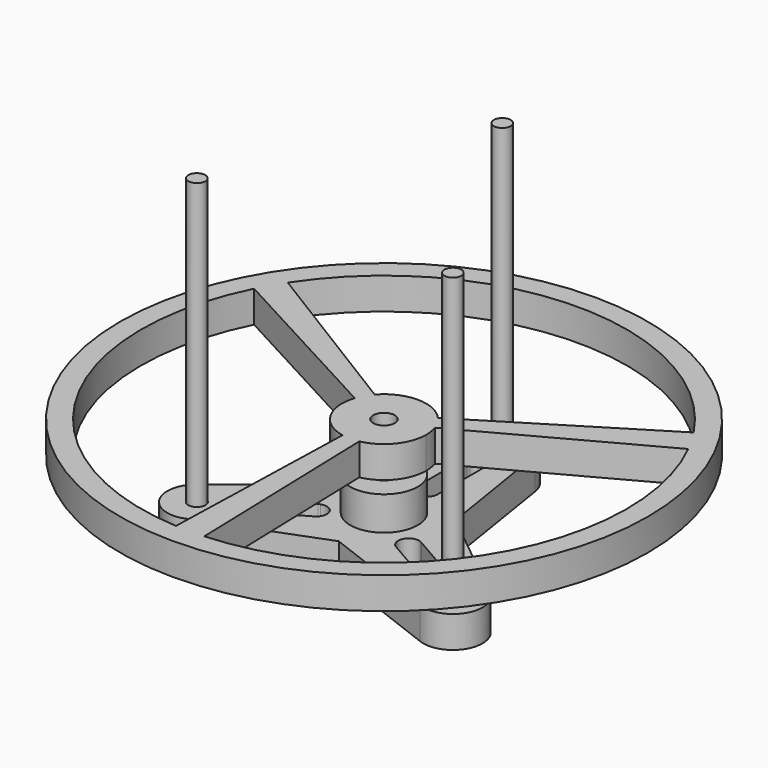
from build123d import *

# Parameters (mm, degrees)
F0_R      = 4
F1_DEPTH  = 150
F2_R      = 4.1
F3_DEPTH  = 15
F5_R      = 125
F6_DEPTH  = 15
F7_D      = 10.2
F9_R      = 16
F10_DEPTH = 16
F11_R     = 5
F12_DEPTH = 15


# Not quite as in the source:
# - a feature names something its author has since deleted; it is built from what else it names


with BuildPart() as f1:
    # F0 (on Top) → F1 (new body)
    with BuildSketch(Plane.XY):
        with Locations((0, 70)):
            Circle(F0_R)
    extrude(amount=F1_DEPTH)


with BuildPart() as f1b:
    # F0 (on Top) → F1, piece 2 (new body)
    with BuildSketch(Plane.XY):
        with Locations((-60.6217782649, -35)):
            Circle(F0_R)
    extrude(amount=F1_DEPTH)


with BuildPart() as f1c:
    # F0 (on Top) → F1, piece 3 (new body)
    with BuildSketch(Plane.XY):
        with Locations((60.6217782649, -35)):
            Circle(F0_R)
    extrude(amount=F1_DEPTH)


with BuildPart() as f3:
    # F2 (on Top) → F3 (new body)
    with BuildSketch(Plane.XY):
        with BuildLine():
            ThreePointArc((-15.7469411811, 19.4173593323), (-10.6083266094, 22.6376546168), (-4.8455068732, 24.5259263462))
            ThreePointArc((-4.8455068732, 24.5259263462), (-4.8928885521, 24.9209603499), (-4.9087158404, 25.3185108304))
            Line((-4.9087158404, 25.3185108304), (-4.9087158404, 55.3185108304))
            ThreePointArc((-4.9087158404, 55.3185108304), (-4.851787509, 56.0709261545), (-4.6822986521, 56.8062105772))
            ThreePointArc((-4.6822986521, 56.8062105772), (-12.0366957637, 62.8503178328), (-13.8260623462, 72.2))
            Line((-13.8260623462, 72.2), (-23.1845919064, 13.3856303782))
            Line((-23.1845919064, 13.3856303782), (-15.7469411811, 19.4173593323))
        make_face()
        with BuildLine():
            ThreePointArc((14, 70), (13.956447844, 71.1034326336), (13.8260623462, 72.2))
            ThreePointArc((13.8260623462, 72.2), (0, 84), (-13.8260623462, 72.2))
            ThreePointArc((-13.8260623462, 72.2), (-12.0366957637, 62.8503178328), (-4.6822986521, 56.8062105772))
            ThreePointArc((-4.6822986521, 56.8062105772), (0.0606919076, 60.3191708855), (4.8473554351, 56.865954725))
            ThreePointArc((4.8473554351, 56.865954725), (11.486143306, 61.9957191482), (14, 70))
        make_face()
        with Locations((0, 70)):
            Circle(F2_R, mode=Mode.SUBTRACT)
        with BuildLine():
            ThreePointArc((5.0236987184, 24.4900480029), (10.6905525136, 22.598939952), (15.7469411811, 19.4173593323))
            Line((15.7469411811, 19.4173593323), (23.1845919064, 13.3856303782))
            Line((23.1845919064, 13.3856303782), (13.8260623462, 72.2))
            ThreePointArc((13.8260623462, 72.2), (13.956447844, 71.1034326336), (14, 70))
            ThreePointArc((14, 70), (11.486143306, 61.9957191482), (4.8473554351, 56.865954725))
            ThreePointArc((4.8473554351, 56.865954725), (5.0210368519, 56.1626662615), (5.0912841596, 55.4416633397))
            Line((5.0912841596, 55.4416633397), (5.0912841596, 25.4416633397))
            ThreePointArc((5.0912841596, 25.4416633397), (5.0802361713, 24.9642402993), (5.0236987184, 24.4900480029))
        make_face()
        with BuildLine():
            ThreePointArc((23.6628287038, -8.0666311267), (24.6634417468, -4.0883543391), (25, 0))
            ThreePointArc((25, 0), (24.9222282929, 1.9704154171), (24.6893970467, 3.9285714286))
            ThreePointArc((24.6893970467, 3.9285714286), (21.6506350946, 12.5), (15.7469411811, 19.4173593323))
            ThreePointArc((15.7469411811, 19.4173593323), (10.6905525136, 22.598939952), (5.0236987184, 24.4900480029))
            ThreePointArc((5.0236987184, 24.4900480029), (0.0738629344, 20.3177855481), (-4.8455068732, 24.5259263462))
            ThreePointArc((-4.8455068732, 24.5259263462), (-10.6083266094, 22.6376546168), (-15.7469411811, 19.4173593323))
            ThreePointArc((-15.7469411811, 19.4173593323), (-21.6506350946, 12.5), (-24.6893970467, 3.9285714286))
            ThreePointArc((-24.6893970467, 3.9285714286), (-24.9165323538, -2.0411799187), (-23.7208530697, -7.8943732904))
            ThreePointArc((-23.7208530697, -7.8943732904), (-17.6326499005, -10.0949255965), (-18.8173218306, -16.4592952196))
            ThreePointArc((-18.8173218306, -16.4592952196), (-14.3006206755, -20.5059076438), (-8.9424558656, -23.3459307609))
            ThreePointArc((-8.9424558656, -23.3459307609), (0, -25), (8.9424558656, -23.3459307609))
            ThreePointArc((8.9424558656, -23.3459307609), (14.2259798402, -20.5577600333), (18.6971543512, -16.5956747126))
            ThreePointArc((18.6971543512, -16.5956747126), (17.5587869661, -10.2228599516), (23.6628287038, -8.0666311267))
        make_face()
        with BuildLine():
            Line((-24.6893970467, 3.9285714286), (-23.1845919064, 13.3856303782))
            Line((-23.1845919064, 13.3856303782), (-69.4400653263, -24.1262787739))
            ThreePointArc((-69.4400653263, -24.1262787739), (-60.5360847426, -21.000262266), (-51.6710391199, -24.2350444145))
            ThreePointArc((-51.6710391199, -24.2350444145), (-51.1488141527, -23.7329876636), (-50.5595309601, -23.3116502498))
            Line((-50.5595309601, -23.3116502498), (-24.5787688465, -8.3116502498))
            ThreePointArc((-24.5787688465, -8.3116502498), (-24.1597843711, -8.0825065681), (-23.7208530697, -7.8943732904))
            ThreePointArc((-23.7208530697, -7.8943732904), (-24.9165323538, -2.0411799187), (-24.6893970467, 3.9285714286))
        make_face()
        with BuildLine():
            ThreePointArc((-69.4400653263, -24.1262787739), (-72.7461339179, -42), (-55.6140029802, -48.0737212261))
            ThreePointArc((-55.6140029802, -48.0737212261), (-49.0868562022, -42.9338246141), (-46.6217782649, -35))
            ThreePointArc((-46.6217782649, -35), (-46.6800730977, -33.723733166), (-46.8544721266, -32.4580948694))
            ThreePointArc((-46.8544721266, -32.4580948694), (-52.2682802758, -30.107024709), (-51.6710391199, -24.2350444145))
            ThreePointArc((-51.6710391199, -24.2350444145), (-60.5360847426, -21.000262266), (-69.4400653263, -24.1262787739))
        make_face()
        with Locations((-60.6217782649, -35)):
            Circle(F2_R, mode=Mode.SUBTRACT)
        with BuildLine():
            Line((0, -26.7712607564), (-8.9424558656, -23.3459307609))
            ThreePointArc((-8.9424558656, -23.3459307609), (-14.3006206755, -20.5059076438), (-18.8173218306, -16.4592952196))
            ThreePointArc((-18.8173218306, -16.4592952196), (-19.1357404737, -16.697845959), (-19.4721156449, -16.910328033))
            Line((-19.4721156449, -16.910328033), (-45.4528777584, -31.910328033))
            ThreePointArc((-45.4528777584, -31.910328033), (-46.132952709, -32.2372343138), (-46.8544721266, -32.4580948694))
            ThreePointArc((-46.8544721266, -32.4580948694), (-46.6800730977, -33.723733166), (-46.6217782649, -35))
            ThreePointArc((-46.6217782649, -35), (-49.0868562022, -42.9338246141), (-55.6140029802, -48.0737212261))
            Line((-55.6140029802, -48.0737212261), (0, -26.7712607564))
        make_face()
        with BuildLine():
            ThreePointArc((19.487484687, -17.1300130899), (19.0795481998, -16.8817337312), (18.6971543512, -16.5956747126))
            ThreePointArc((18.6971543512, -16.5956747126), (14.2259798402, -20.5577600333), (8.9424558656, -23.3459307609))
            Line((8.9424558656, -23.3459307609), (0, -26.7712607564))
            Line((0, -26.7712607564), (55.6140029802, -48.0737212261))
            ThreePointArc((55.6140029802, -48.0737212261), (48.4548029798, -41.9256560998), (46.8236836847, -32.6309103105))
            ThreePointArc((46.8236836847, -32.6309103105), (46.1277773008, -32.4296785979), (45.4682468005, -32.1300130899))
            Line((45.4682468005, -32.1300130899), (19.487484687, -17.1300130899))
        make_face()
        with BuildLine():
            ThreePointArc((24.6893970467, 3.9285714286), (24.9222282929, 1.9704154171), (25, 0))
            ThreePointArc((25, 0), (24.6634417468, -4.0883543391), (23.6628287038, -8.0666311267))
            ThreePointArc((23.6628287038, -8.0666311267), (24.0286290258, -8.2231143909), (24.3808314853, -8.4081827974))
            Line((24.3808314853, -8.4081827974), (50.3615935989, -23.4081827974))
            ThreePointArc((50.3615935989, -23.4081827974), (50.984740218, -23.8336918407), (51.5367707787, -24.3481157078))
            ThreePointArc((51.5367707787, -24.3481157078), (60.448319761, -21.0010746074), (69.4400653263, -24.1262787739))
            Line((69.4400653263, -24.1262787739), (23.1845919064, 13.3856303782))
            Line((23.1845919064, 13.3856303782), (24.6893970467, 3.9285714286))
        make_face()
        with BuildLine():
            ThreePointArc((74.6217782649, -35), (73.2601329612, -28.97737677), (69.4400653263, -24.1262787739))
            ThreePointArc((69.4400653263, -24.1262787739), (60.448319761, -21.0010746074), (51.5367707787, -24.3481157078))
            ThreePointArc((51.5367707787, -24.3481157078), (52.2075883683, -30.2121461765), (46.8236836847, -32.6309103105))
            ThreePointArc((46.8236836847, -32.6309103105), (48.4548029798, -41.9256560998), (55.6140029802, -48.0737212261))
            ThreePointArc((55.6140029802, -48.0737212261), (68.555602879, -46.5349220627), (74.6217782649, -35))
        make_face()
        with Locations((60.6217782649, -35)):
            Circle(F2_R, mode=Mode.SUBTRACT)
        with BuildLine():
            ThreePointArc((15.7469411811, 19.4173593323), (21.6506350946, 12.5), (24.6893970467, 3.9285714286))
            Line((24.6893970467, 3.9285714286), (23.1845919064, 13.3856303782))
            Line((23.1845919064, 13.3856303782), (15.7469411811, 19.4173593323))
        make_face()
        with BuildLine():
            ThreePointArc((-24.6893970467, 3.9285714286), (-21.6506350946, 12.5), (-15.7469411811, 19.4173593323))
            Line((-15.7469411811, 19.4173593323), (-23.1845919064, 13.3856303782))
            Line((-23.1845919064, 13.3856303782), (-24.6893970467, 3.9285714286))
        make_face()
        with BuildLine():
            Line((0, -26.7712607564), (8.9424558656, -23.3459307609))
            ThreePointArc((8.9424558656, -23.3459307609), (0, -25), (-8.9424558656, -23.3459307609))
            Line((-8.9424558656, -23.3459307609), (0, -26.7712607564))
        make_face()
    extrude(amount=F3_DEPTH)


with BuildPart() as f6:
    # F5 (on offset) → F6 (new body)
    with BuildSketch(Plane.XY.offset(40)):
        Circle(F5_R)
        with BuildLine():
            ThreePointArc((102.7583822566, 51.6305614534), (111.8977523445, 26.5309822706), (115, 0))
            ThreePointArc((115, 0), (83.6577855811, -78.9073818579), (6.7152189274, -114.8037709954))
            ThreePointArc((6.7152189274, -114.8037709954), (0.0247447273, -114.9999973378), (-6.665813298, -114.8066502128))
            ThreePointArc((-6.665813298, -114.8066502128), (-99.5805467661, -57.5214282313), (-102.7805915959, 51.5863353146))
            ThreePointArc((-102.7805915959, 51.5863353146), (-99.6052914933, 57.4785691065), (-96.0925689586, 63.1760887593))
            ThreePointArc((-96.0925689586, 63.1760887593), (-0.0247447273, 114.9999973378), (96.0653726685, 63.2174356808))
            ThreePointArc((96.0653726685, 63.2174356808), (99.5805467661, 57.5214282313), (102.7583822566, 51.6305614534))
        make_face(mode=Mode.SUBTRACT)
        with BuildLine():
            Line((-14.9932737383, 13.2363795129), (-96.0925689586, 63.1760887593))
            ThreePointArc((-96.0925689586, 63.1760887593), (-99.6052914933, 57.4785691065), (-102.7805915959, 51.5863353146))
            Line((-102.7805915959, 51.5863353146), (-18.9593623085, 6.3673056198))
            ThreePointArc((-18.9593623085, 6.3673056198), (-17.3202603233, 10.0004291074), (-14.9932737383, 13.2363795129))
        make_face()
        with BuildLine():
            Line((18.9596777814, 6.3663661868), (102.7583822566, 51.6305614534))
            ThreePointArc((102.7583822566, 51.6305614534), (99.5805467661, 57.5214282313), (96.0653726685, 63.2174356808))
            Line((96.0653726685, 63.2174356808), (14.9939295747, 13.2356365888))
            ThreePointArc((14.9939295747, 13.2356365888), (17.3207558174, 9.9995708864), (18.9596777814, 6.3663661868))
        make_face()
        with BuildLine():
            ThreePointArc((-6.665813298, -114.8066502128), (0.0247447273, -114.9999973378), (6.7152189274, -114.8037709954))
            Line((6.7152189274, -114.8037709954), (3.9654327338, -19.6029422086))
            ThreePointArc((3.9654327338, -19.6029422086), (-0.0004954941, -19.9999999939), (-3.9664040432, -19.6027456997))
            Line((-3.9664040432, -19.6027456997), (-6.665813298, -114.8066502128))
        make_face()
        with BuildLine():
            ThreePointArc((20, 0), (19.7382060435, 3.2254026393), (18.9596777814, 6.3663661868))
            ThreePointArc((18.9596777814, 6.3663661868), (17.3207558174, 9.9995708864), (14.9939295747, 13.2356365888))
            ThreePointArc((14.9939295747, 13.2356365888), (0.0004954941, 19.9999999939), (-14.9932737383, 13.2363795129))
            ThreePointArc((-14.9932737383, 13.2363795129), (-17.3202603233, 10.0004291074), (-18.9593623085, 6.3673056198))
            ThreePointArc((-18.9593623085, 6.3673056198), (-17.3207558174, -9.9995708864), (-3.9664040432, -19.6027456997))
            ThreePointArc((-3.9664040432, -19.6027456997), (-0.0004954941, -19.9999999939), (3.9654327338, -19.6029422086))
            ThreePointArc((3.9654327338, -19.6029422086), (15.4807728275, -12.6627671803), (20, 0))
        make_face()
    extrude(amount=F6_DEPTH)

    # F7 (through all)
    with Locations(Plane(origin=(0, 0, 0), x_dir=(1, 0, 0), z_dir=(0, 0, -1))):
        with Locations((0, 0)):
            Hole(F7_D / 2)


with BuildPart() as f10:
    # F9 (on offset) → F10 (new body)
    with BuildSketch(Plane.XY.offset(16)):
        Circle(F9_R)
    extrude(amount=F10_DEPTH)

    # F11 (on face) → F12 (join)
    with BuildSketch(Plane.XY.offset(32)):
        Circle(F11_R)
    extrude(amount=F12_DEPTH)


solid = Compound([f1.part, f1b.part, f1c.part, f3.part, f6.part, f10.part])
